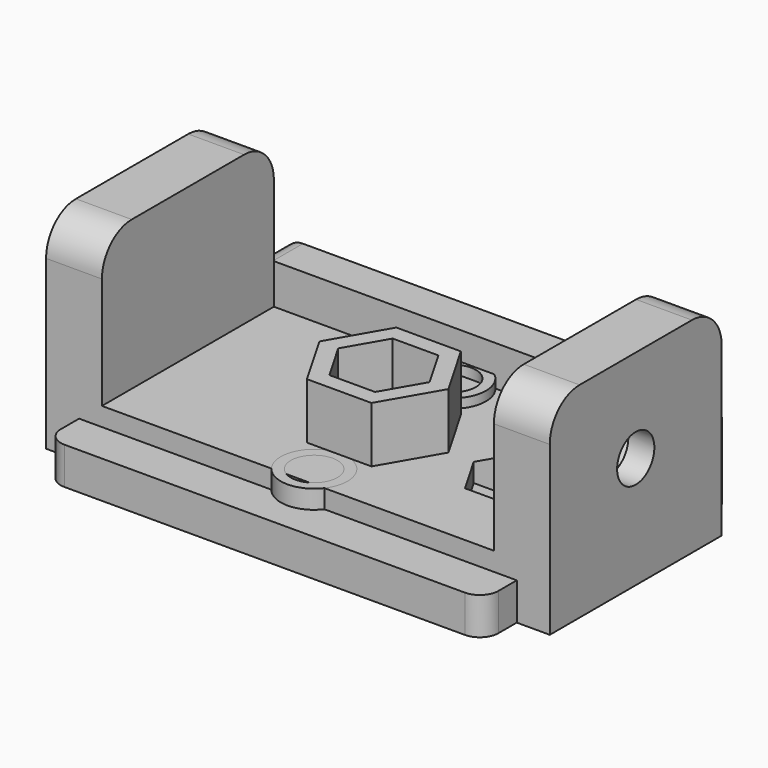
from build123d import *

# Parameters (mm, degrees)
F0_W      = 23.5
F0_H      = 14
F0_W_2    = 19.5
F0_H_2    = 2.5
F1_DEPTH  = 2
F0_H_3    = 2
F2_DEPTH  = 5
F3_R      = 1
F4_W      = 21.0458148676
F4_H      = 11.5377975056
F5_DEPTH  = 3
F4_W_2    = 3
F6_DEPTH  = 11
F4_R      = 1.25
F8_DEPTH  = 1.4
F7_R      = 1.25
F9_DEPTH  = 3.001
F10_DEPTH = 1.6
F11_R     = 2
F12_R     = 1.7907796981
F12_R_2   = 1.25
F13_DEPTH = 3.5
F14_DEPTH = 3.25
F15_DEPTH = 3
F16_R     = 1.5
F17_DEPTH = 3
F18_DEPTH = 6


with BuildPart() as f1:
    # F0 (on Top) → F1 (new body)
    with BuildSketch(Plane.XY):
        with Locations((0, -1)):
            Rectangle(F0_W, F0_H)
        with Locations((0, 1.25)):
            Rectangle(F0_W_2, F0_H_2, mode=Mode.SUBTRACT)
    extrude(amount=F1_DEPTH)

    # F0 (on Top) → F2 (join)
    with BuildSketch(Plane.XY):
        with Locations((0, 7)):
            Rectangle(F0_W, F0_H_3)
    extrude(amount=F2_DEPTH)

    # F3
    f3_edges = [f1.edges().sort_by_distance(p)[0] for p in [
        (-9.75, 2.5, 1),
        (-9.75, 0, 1),
        (9.75, 2.5, 1),
        (9.75, 0, 1),
        (11.75, 7, 5),
        (-11.75, 7, 5),
        (-11.75, -8, 1),
        (11.75, -8, 1),
    ]]
    fillet(f3_edges, radius=F3_R)


with BuildPart() as f5:
    # F4 (on Top) → F5 (new body)
    with BuildSketch(Plane.XY):
        Rectangle(F4_W, F4_H)
        Polygon((9.6710080965, 0), (8.4585725312, -2.1), (6.0337014006, -2.1), (4.8212658353, 0), (6.0337014006, 2.1), (8.4585725312, 2.1), align=None, mode=Mode.SUBTRACT)
    extrude(amount=F5_DEPTH)

    # F4 (on Top) → F6 (join)
    with BuildSketch(Plane.XY):
        with Locations((-12.0229074338, 0)):
            Rectangle(F4_W_2, F4_H)
        with Locations((12.0229074338, 0)):
            Rectangle(F4_W_2, F4_H)
    extrude(amount=F6_DEPTH)

    # F4 (on Top) → F8 (join)
    with BuildSketch(Plane.XY):
        Polygon((6.0337014006, -2.1), (8.4585725312, -2.1), (9.6710080965, 0), (8.4585725312, 2.1), (6.0337014006, 2.1), (4.8212658353, 0), align=None)
        with Locations((7.2461369659, 0)):
            Circle(F4_R, mode=Mode.SUBTRACT)
    extrude(amount=F8_DEPTH)

    # F7 (on face) → F9 (cut, through all)
    with BuildSketch(Plane(origin=(10.5229074338, 0, 0), x_dir=(0, -1, 0), z_dir=(-1, 0, 0))):
        with Locations((0, 6)):
            Circle(F7_R)
    extrude(amount=-F9_DEPTH, mode=Mode.SUBTRACT)

    # F7 (on face) → F10 (cut)
    with BuildSketch(Plane(origin=(10.5229074338, 0, 0), x_dir=(0, -1, 0), z_dir=(-1, 0, 0))):
        Polygon((-1.2124355653, 3.9), (1.2124355653, 3.9), (2.4248711306, 6), (1.2124355653, 8.1), (-1.2124355653, 8.1), (-2.4248711306, 6), align=None)
        with Locations((0, 6)):
            Circle(F7_R, mode=Mode.SUBTRACT)
    extrude(amount=-F10_DEPTH, mode=Mode.SUBTRACT)

    # F11
    f11_edges = [f5.edges().sort_by_distance(p)[0] for p in [
        (-12.022907, -5.768899, 11),
        (12.022907, -5.768899, 11),
        (12.022907, 5.768899, 11),
        (-12.022907, 5.768899, 11),
    ]]
    fillet(f11_edges, radius=F11_R)


with BuildPart() as f13:
    # F12 (on Top) → F13 (new body)
    with BuildSketch(Plane.XY):
        with Locations((0, 4.6143797226)):
            Circle(F12_R)
        with Locations((0, 4.6143797226)):
            Circle(F12_R_2, mode=Mode.SUBTRACT)
    extrude(amount=F13_DEPTH)


with BuildPart() as f14:
    # F12 (on Top) → F14 (new body)
    with BuildSketch(Plane.XY):
        Circle(F12_R)
        Circle(F12_R_2, mode=Mode.SUBTRACT)
    extrude(amount=F14_DEPTH)


with BuildPart() as f15:
    # F12 (on Top) → F15 (new body)
    with BuildSketch(Plane.XY):
        with Locations((0, -4.6819411218)):
            Circle(F12_R)
        with Locations((0, -4.6819411218)):
            Circle(F12_R_2, mode=Mode.SUBTRACT)
    extrude(amount=F15_DEPTH)


with BuildPart() as f17:
    # F16 (on Top) → F17 (new body)
    with BuildSketch(Plane.XY):
        Polygon((-1.7320508076, 3), (-3.4641016151, 0), (-1.7320508076, -3), (1.7320508076, -3), (3.4641016151, 0), (1.7320508076, 3), align=None)
        Polygon((-1.226869322, -2.125), (-2.4537386441, 0), (-1.226869322, 2.125), (1.226869322, 2.125), (2.4537386441, 0), (1.226869322, -2.125), align=None, mode=Mode.SUBTRACT)
        Polygon((-1.226869322, 2.125), (-2.4537386441, 0), (-1.226869322, -2.125), (1.226869322, -2.125), (2.4537386441, 0), (1.226869322, 2.125), align=None)
        Circle(F16_R, mode=Mode.SUBTRACT)
    extrude(amount=F17_DEPTH)

    # F16 (on Top) → F18 (join)
    with BuildSketch(Plane.XY):
        Polygon((-1.7320508076, 3), (-3.4641016151, 0), (-1.7320508076, -3), (1.7320508076, -3), (3.4641016151, 0), (1.7320508076, 3), align=None)
        Polygon((-1.226869322, -2.125), (-2.4537386441, 0), (-1.226869322, 2.125), (1.226869322, 2.125), (2.4537386441, 0), (1.226869322, -2.125), align=None, mode=Mode.SUBTRACT)
    extrude(amount=F18_DEPTH)


solid = Compound([f1.part, f5.part, f13.part, f14.part, f15.part, f17.part])
